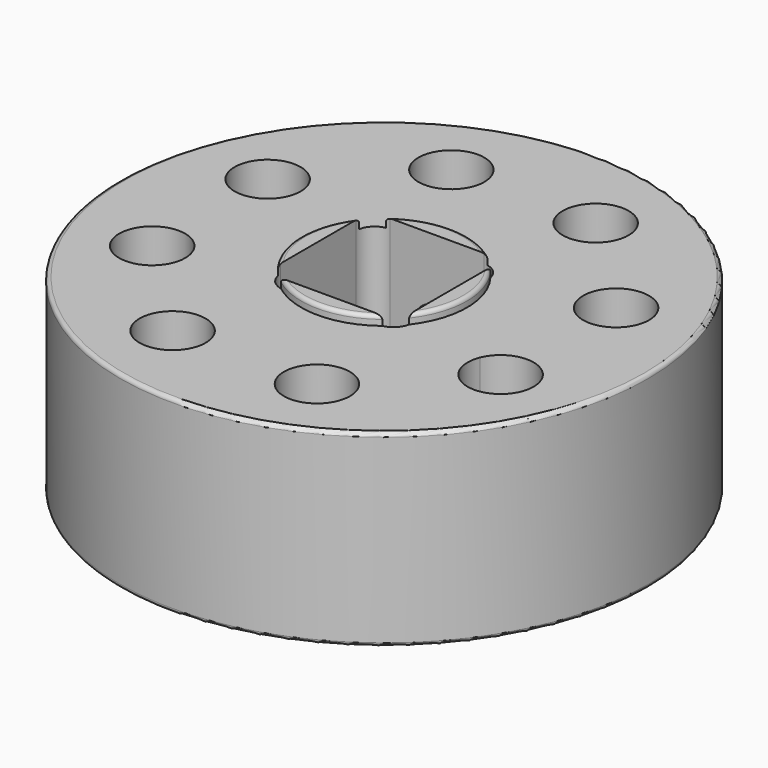
from build123d import *

# Parameters (mm, degrees)
F0_R          = 14
F1_DEPTH      = 10
F2_R          = 4.4
F3_DEPTH      = 0.5
F4_W          = 7
F4_H          = 7
F5_DEPTH      = 8
F6_R          = 2.15
F7_DEPTH      = 2.5
F8_R          = 1.75
F9_DEPTH      = 10
F10_R         = 1.25
F11_DEPTH     = 25
F12_R         = 1.25
F13_DEPTH     = 25
F14_T1_DEPTH  = 10
F14_T6_DEPTH  = 12.5
F14_S7_R      = 4.4
F14_T8_DEPTH  = 8
F14_T13_DEPTH = 12.5
F14_S14_R     = 4.4
F14_T15_DEPTH = 8
F14_T20_DEPTH = 12.5
F14_S21_R     = 4.4
F14_T22_DEPTH = 8
F14_T27_DEPTH = 12.5
F14_S28_R     = 4.4
F14_T29_DEPTH = 8
F15_R         = 0.2


# Not quite as in the source:
# - a fillet or chamfer that OpenCascade refuses, or shapes differently, is made with other operations: its cross-section is extruded or revolved along the edge and cut away or added
# - a feature names something its author has since deleted; it is built from what else it names


with BuildPart() as f1:
    # F0 (on Top) → F1 (new body)
    with BuildSketch(Plane.XY):
        Circle(F0_R)
    extrude(amount=F1_DEPTH)

    # F2 (on face) → F3 (join)
    with BuildSketch(Plane.XY.offset(10)):
        Circle(F2_R)
    extrude(amount=F3_DEPTH)

    # F4 (on face) → F5 (cut)
    with BuildSketch(Plane.XY.offset(10.5)):
        Rectangle(F4_W, F4_H)
    extrude(amount=-F5_DEPTH, mode=Mode.SUBTRACT)

    # F6 (on face) → F7 (cut, through all)
    with BuildSketch(Plane(origin=(0, 0, 0), x_dir=(1, 0, 0), z_dir=(0, 0, -1))):
        Circle(F6_R)
    extrude(amount=-F7_DEPTH, mode=Mode.SUBTRACT)

    # F8 (on face) → F9 (cut, through all)
    with BuildSketch(Plane(origin=(0, 0, 0), x_dir=(1, 0, 0), z_dir=(0, 0, -1))):
        with BuildLine():
            ThreePointArc((7.6220061432, 3.157138317), (9.5802033886, 2.1104600829), (10.9887953251, 3.8268343237))
            ThreePointArc((10.9887953251, 3.8268343237), (8.8973872616, 5.5432085644), (7.6220061432, 3.157138317))
        make_face()
        with Locations((3.8268343237, 9.2387953251)):
            Circle(F8_R)
        with Locations((-3.8268343237, 9.2387953251)):
            Circle(F8_R)
        with Locations((-9.2387953251, 3.8268343237)):
            Circle(F8_R)
        with Locations((-9.2387953251, -3.8268343237)):
            Circle(F8_R)
        with Locations((-3.8268343237, -9.2387953251)):
            Circle(F8_R)
        with Locations((3.8268343237, -9.2387953251)):
            Circle(F8_R)
        with Locations((9.2387953251, -3.8268343237)):
            Circle(F8_R)
    extrude(amount=-F9_DEPTH, mode=Mode.SUBTRACT)

    # F10 (on Front) → F11 (cut)
    with BuildSketch(Plane.XZ):
        with Locations((0, 6)):
            Circle(F10_R)
    extrude(amount=-F11_DEPTH, mode=Mode.SUBTRACT)

    # F12 (on Right) → F13 (cut)
    with BuildSketch(Plane.YZ):
        with Locations((0, 6)):
            Circle(F12_R)
    extrude(amount=-F13_DEPTH, mode=Mode.SUBTRACT)

    # F14: fillet of radius 1 on 4 edges, made by hand

    # F14_s2 → F14_t1 (join)
    with BuildSketch(Plane.XY):
        with BuildLine():
            ThreePointArc((-2.5, -3.5), (-3.2071067812, -3.2071067812), (-3.5, -2.5))
            Line((-3.5, -2.5), (-3.5, -3.5))
            Line((-3.5, -3.5), (-2.5, -3.5))
        make_face()
        with BuildLine():
            ThreePointArc((3.5, -2.5), (3.2071067812, -3.2071067812), (2.5, -3.5))
            Line((2.5, -3.5), (3.5, -3.5))
            Line((3.5, -3.5), (3.5, -2.5))
        make_face()
        with BuildLine():
            ThreePointArc((3.5, 2.5), (3.2071067812, 3.2071067812), (2.5, 3.5))
            Line((2.5, 3.5), (3.5, 3.5))
            Line((3.5, 3.5), (3.5, 2.5))
        make_face()
        with BuildLine():
            ThreePointArc((-2.5, 3.5), (-3.2071067812, 3.2071067812), (-3.5, 2.5))
            Line((-3.5, 2.5), (-3.5, 3.5))
            Line((-3.5, 3.5), (-2.5, 3.5))
        make_face()
    extrude(amount=F14_T1_DEPTH)


with BuildPart() as f14_tool4:
    # F14_s5 → F14_t6 (new body)
    with BuildSketch(Plane.XY.offset(12.5)):
        with BuildLine():
            ThreePointArc((-2.5, -3.5), (-3.2071067812, -3.2071067812), (-3.5, -2.5))
            Line((-3.5, -2.5), (-3.5, -3.5))
            Line((-3.5, -3.5), (-2.5, -3.5))
        make_face()
    extrude(amount=-F14_T6_DEPTH)

    # F14_s7 → F14_t8 (intersect, symmetric)
    with BuildSketch(Plane.XY.offset(6.2)):
        Circle(F14_S7_R)
    extrude(amount=F14_T8_DEPTH, both=True, mode=Mode.INTERSECT)

    split(bisect_by=Plane.XY.offset(10.5), keep=Keep.BOTTOM)


with BuildPart() as f1_1:
    add(f1.part)

    # F14_t3: union F14_tool4
    add(f14_tool4.part)


with BuildPart() as f14_tool11:
    # F14_s12 → F14_t13 (new body)
    with BuildSketch(Plane.XY.offset(12.5)):
        with BuildLine():
            ThreePointArc((3.5, -2.5), (3.2071067812, -3.2071067812), (2.5, -3.5))
            Line((2.5, -3.5), (3.5, -3.5))
            Line((3.5, -3.5), (3.5, -2.5))
        make_face()
    extrude(amount=-F14_T13_DEPTH)

    # F14_s14 → F14_t15 (intersect, symmetric)
    with BuildSketch(Plane.XY.offset(6.2)):
        Circle(F14_S14_R)
    extrude(amount=F14_T15_DEPTH, both=True, mode=Mode.INTERSECT)

    split(bisect_by=Plane.XY.offset(10.5), keep=Keep.BOTTOM)


with BuildPart() as f1_2:
    add(f1_1.part)

    # F14_t10: union F14_tool11
    add(f14_tool11.part)


with BuildPart() as f14_tool18:
    # F14_s19 → F14_t20 (new body)
    with BuildSketch(Plane.XY.offset(12.5)):
        with BuildLine():
            ThreePointArc((3.5, 2.5), (3.2071067812, 3.2071067812), (2.5, 3.5))
            Line((2.5, 3.5), (3.5, 3.5))
            Line((3.5, 3.5), (3.5, 2.5))
        make_face()
    extrude(amount=-F14_T20_DEPTH)

    # F14_s21 → F14_t22 (intersect, symmetric)
    with BuildSketch(Plane.XY.offset(6.2)):
        Circle(F14_S21_R)
    extrude(amount=F14_T22_DEPTH, both=True, mode=Mode.INTERSECT)

    split(bisect_by=Plane.XY.offset(10.5), keep=Keep.BOTTOM)


with BuildPart() as f1_3:
    add(f1_2.part)

    # F14_t17: union F14_tool18
    add(f14_tool18.part)


with BuildPart() as f14_tool25:
    # F14_s26 → F14_t27 (new body)
    with BuildSketch(Plane.XY.offset(12.5)):
        with BuildLine():
            ThreePointArc((-2.5, 3.5), (-3.2071067812, 3.2071067812), (-3.5, 2.5))
            Line((-3.5, 2.5), (-3.5, 3.5))
            Line((-3.5, 3.5), (-2.5, 3.5))
        make_face()
    extrude(amount=-F14_T27_DEPTH)

    # F14_s28 → F14_t29 (intersect, symmetric)
    with BuildSketch(Plane.XY.offset(6.2)):
        Circle(F14_S28_R)
    extrude(amount=F14_T29_DEPTH, both=True, mode=Mode.INTERSECT)

    split(bisect_by=Plane.XY.offset(10.5), keep=Keep.BOTTOM)


with BuildPart() as f1_4:
    add(f1_3.part)

    # F14_t24: union F14_tool25
    add(f14_tool25.part)

    # F15
    f15_edges = [f1_4.edges().sort_by_distance(p)[0] for p in [
        (-14, 0, 10),
        (-14, 0, 0),
        (-4.4, 0, 10.5),
        (0, -4.4, 10.5),
        (4.4, 0, 10.5),
        (0, 4.4, 10.5),
    ]]
    fillet(f15_edges, radius=F15_R)


solid = f1_4.part
